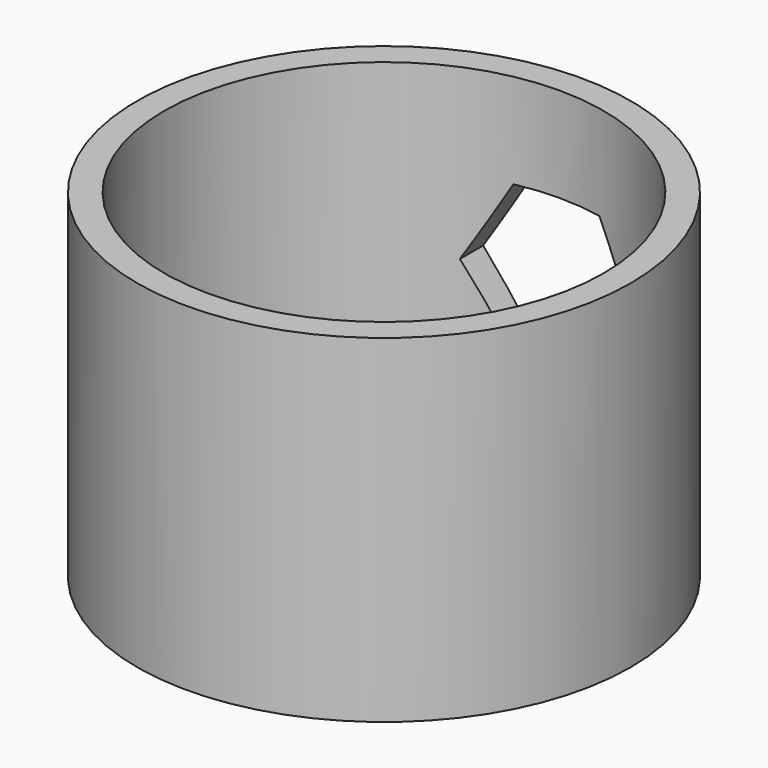
from build123d import *

# Parameters (mm, degrees)
F0_R     = 36.5
F0_R_2   = 32.5
F1_DEPTH = 25
F3_DEPTH = 40


# Not quite as in the source:
# - a feature names something its author has since deleted; it is built from what else it names


with BuildPart() as f1:
    # F0 (on Top) → F1 (new body, symmetric)
    with BuildSketch(Plane.XY):
        Circle(F0_R)
        Circle(F0_R_2, mode=Mode.SUBTRACT)
    extrude(amount=F1_DEPTH, both=True)

    # F2 (on Front) → F3 (cut)
    with BuildSketch(Plane.XZ):
        Polygon((-6.3508529611, -11), (6.3508529611, -11), (12.7017059222, 0), (6.3508529611, 11), (-6.3508529611, 11), (-12.7017059222, 0), align=None)
    extrude(amount=-F3_DEPTH, mode=Mode.SUBTRACT)


solid = f1.part
